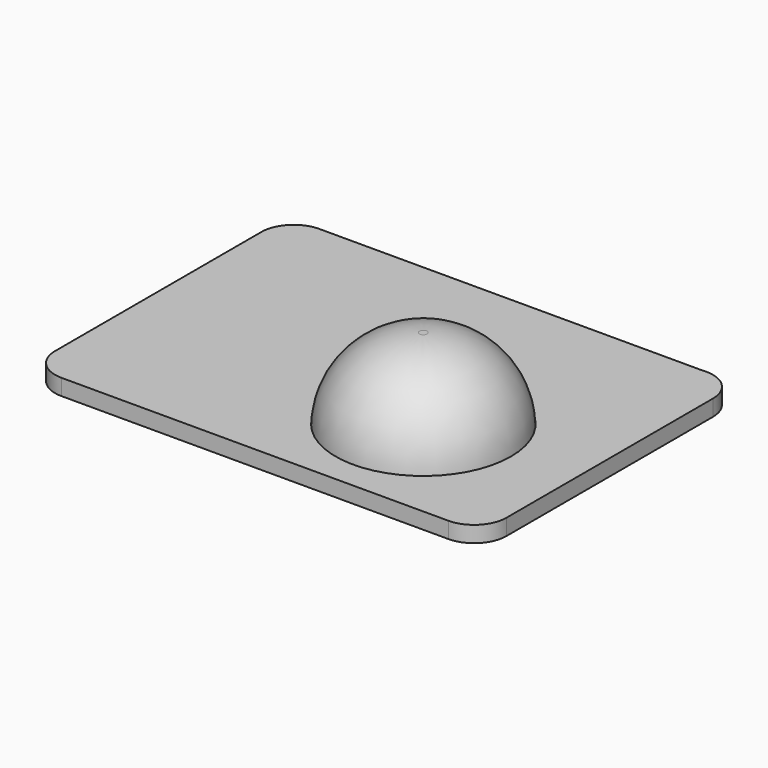
from build123d import *

# Parameters (mm, degrees)
F0_R     = 34.544
F1_DEPTH = 38.1
F2_R     = 33.02
F4_DEPTH = 6.35


# Not quite as in the source:
# - the program builds the solid bodies; features that only make, move or delete a surface that nothing else refers to are left out


with BuildPart() as f1:
    # F0 (on Top) → F1 (new body)
    with BuildSketch(Plane.XY):
        with Locations((29.9727506936, -18.0700458586)):
            Circle(F0_R)
    extrude(amount=F1_DEPTH)

    # F2
    f2_edges = [f1.edges().sort_by_distance(p)[0] for p in [
        (-4.571249, -18.070046, 38.1),
    ]]
    fillet(f2_edges, radius=F2_R)

    # F0 (on Top) → F4 (join)
    with BuildSketch(Plane.XY):
        with BuildLine():
            Line((-76.2, -63.5), (76.2, -63.5))
            ThreePointArc((76.2, -63.5), (85.1802561211, -59.7802561211), (88.9, -50.8))
            Line((88.9, -50.8), (88.9, 50.8837117301))
            ThreePointArc((88.9, 50.8837117301), (84.6499025139, 60.364700471), (74.7442287394, 63.500000013))
            Line((74.7442287394, 63.500000013), (-31.496, 63.500000013))
            Line((-31.496, 63.500000013), (-51.816, 63.5))
            Line((-51.816, 63.5), (-76.2, 63.5))
            ThreePointArc((-76.2, 63.5), (-85.1802561211, 59.7802561211), (-88.9, 50.8))
            Line((-88.9, 50.8), (-88.9, -50.8))
            ThreePointArc((-88.9, -50.8), (-85.1802561211, -59.7802561211), (-76.2, -63.5))
        make_face()
        with Locations((29.9727506936, -18.0700458586)):
            Circle(F0_R, mode=Mode.SUBTRACT)
    extrude(amount=F4_DEPTH)


solid = f1.part
